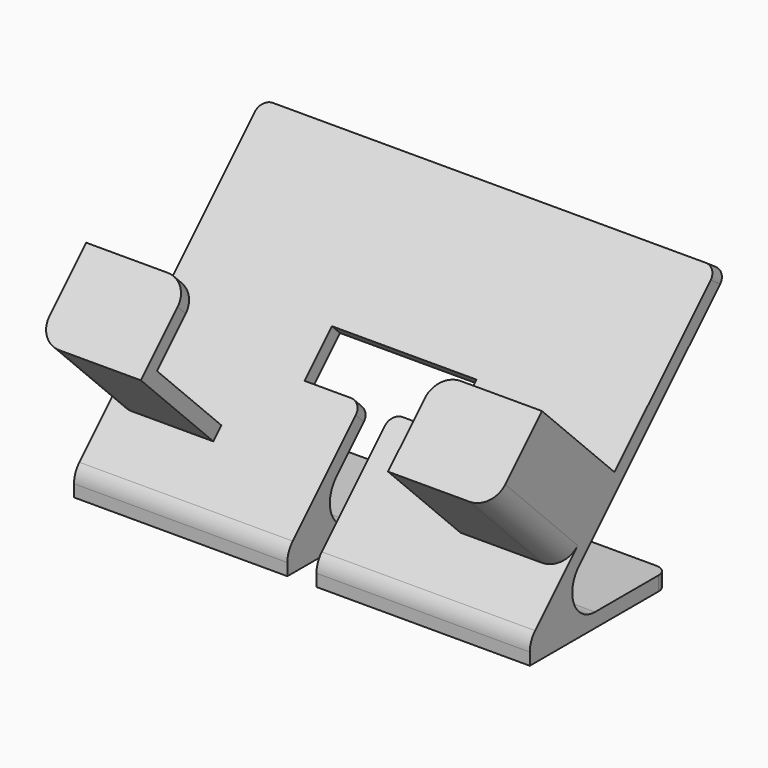
from build123d import *

# Parameters (mm, degrees)
F1_DEPTH = 50.8
F3_DEPTH = 25.4
F4_W     = 16.1045007408
F4_H     = 10.7811614871
F5_DEPTH = 3.175
F6_W     = 3.2399867196
F6_H     = 27.9691088945
F7_REACH = 85.1871733106
F8_W     = 23.2520068914
F8_H     = 19.5576284379
F9_DEPTH = 3.175
F10_R    = 5.08
F11_R    = 2.54


with BuildPart() as f1:
    # F0 (on Right) → F1 (new body)
    with BuildSketch(Plane.YZ):
        with BuildLine():
            Line((0, 0), (38.4632237256, 0))
            Line((38.4632237256, 0), (38.4632237256, 3.175))
            Line((38.4632237256, 3.175), (18.1845425574, 3.175))
            ThreePointArc((18.1845425574, 3.175), (12.3179075259, 7.0949602045), (13.6944144968, 14.0151280605))
            Line((13.6944144968, 14.0151280605), (54.8708899793, 55.191603543))
            Line((54.8708899793, 55.191603543), (52.2191855315, 57.0300271557))
            Line((52.2191855315, 57.0300271557), (0, 4.8108416242))
            Line((0, 4.8108416242), (0, 0))
        make_face()
    extrude(amount=F1_DEPTH)

    # F2 (on face) → F3 (join)
    with BuildSketch(Plane(origin=(0, -2.4054208121, 2.4054208121), x_dir=(1, 0, 0), z_dir=(0, -0.7071067812, 0.7071067812))):
        Polygon((27.5479931086, 17.2171894163), (50.8, 17.2171894163), (50.8, 36.7748178542), (47.625, 36.7748178542), (47.625, 20.3921894163), (27.5479931086, 20.3921894163), align=None)
    extrude(amount=F3_DEPTH)

    # F4 (on face) → F5 (cut, through all)
    with BuildSketch(Plane(origin=(0, -2.4054208121, 2.4054208121), x_dir=(1, 0, 0), z_dir=(0, -0.7071067812, 0.7071067812))):
        with Locations((8.0522503704, 38.3052378893)):
            Rectangle(F4_W, F4_H)
    extrude(amount=-F5_DEPTH, mode=Mode.SUBTRACT)

    f7_end = Plane(origin=(8.0522503704, 21.9912884712, 24.5570660652), x_dir=(0, 0.7071067812, -0.7071067812), z_dir=(0, 0.7071067812, 0.7071067812))
    # F6 (on Top) → F7 (cut, up to a plane its end follows)
    with BuildSketch(Plane.XY):
        with Locations((1.6199933598, 13.9845544472)):
            Rectangle(F6_W, F6_H)
    f7_long = extrude(amount=F7_REACH, mode=Mode.PRIVATE)
    add(split(f7_long, bisect_by=f7_end, keep=Keep.BOTTOM, mode=Mode.PRIVATE), mode=Mode.SUBTRACT)

    # F8 (on face) → F9 (join)
    with BuildSketch(Plane(origin=(0, -20.3659330543, 20.3659330543), x_dir=(1, 0, 0), z_dir=(0, -0.7071067812, 0.7071067812))):
        with Locations((39.1739965543, 26.9960036352)):
            Rectangle(F8_W, F8_H)
    extrude(amount=F9_DEPTH)

    # F10
    f10_edges = [f1.edges().sort_by_distance(p)[0] for p in [
        (27.019993, 0, 4.810842),
        (50.8, -0.333818, 24.6826),
        (27.547993, 4.515258, 47.492188),
    ]]
    fillet(f10_edges, radius=F10_R)

    # F11
    f11_edges = [f1.edges().sort_by_distance(p)[0] for p in [
        (50.8, 53.545038, 56.110815),
        (50.8, 38.463224, 1.5875),
        (3.239987, 21.991288, 24.557066),
    ]]
    fillet(f11_edges, radius=F11_R)

    # F12: F1 across plane


with BuildPart() as f1_1:
    add(f1.part)
    add(f1.part.mirror(Plane.YZ))


solid = f1_1.part
